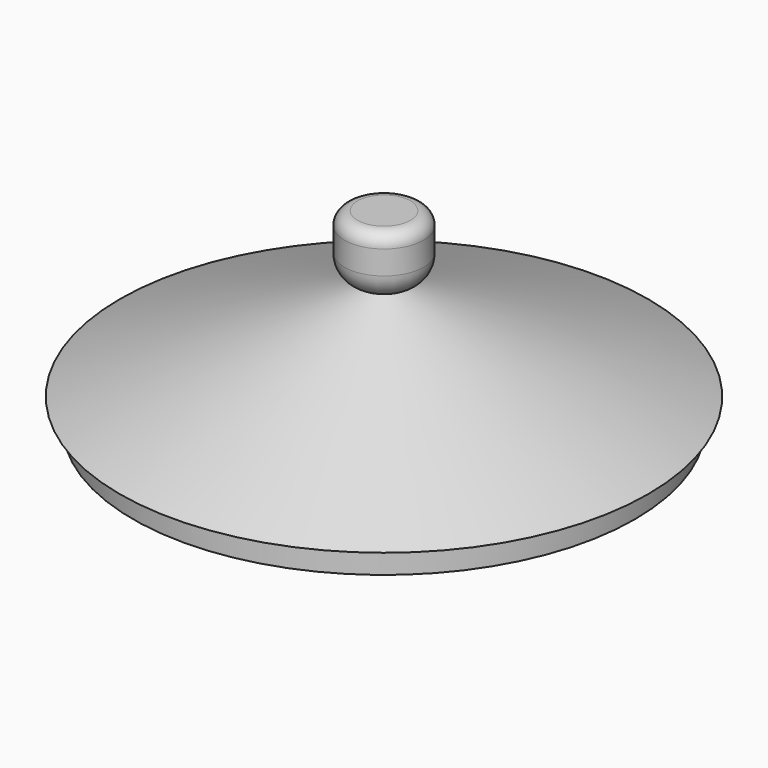
from build123d import *

# Parameters (mm, degrees)
F2_R      = 2.5
F0_R      = 50
F5_R      = 7.5
F6_DEPTH  = 12
F7_R      = 2.5
F8_R      = 4.99999
F9_R      = 47.5
F10_DEPTH = 5


# Not quite as in the source:
# - a fillet or chamfer is up to 0.001 mm smaller than in the source, because OpenCascade refuses the exact size


with BuildPart() as f3:
    # F2 (on offset) → F3 section 0
    with BuildSketch(Plane.XY.offset(19)):
        Circle(F2_R)
    # F0 (on Top) → F3 section 1
    with BuildSketch(Plane.XY):
        Circle(F0_R)
    loft()

    # F5 (on offset) → F6 (join)
    with BuildSketch(Plane.XY.offset(19)):
        Circle(F5_R)
    extrude(amount=F6_DEPTH)

    # F7
    f7_edges = [f3.edges().sort_by_distance(p)[0] for p in [
        (-7.5, 0, 31),
    ]]
    fillet(f7_edges, radius=F7_R)

    # F8 (radius 5 in the source; OpenCascade refuses exactly that, so slightly less here)
    f8_edges = [f3.edges().sort_by_distance(p)[0] for p in [
        (-7.5, 0, 19),
    ]]
    fillet(f8_edges, radius=F8_R)

    # F9 (on Top) → F10 (join)
    with BuildSketch(Plane.XY):
        Circle(F9_R)
    extrude(amount=-F10_DEPTH)


with BuildPart() as f4:
    # F2 (on offset) → F4 section 0
    with BuildSketch(Plane.XY.offset(19)):
        Circle(F2_R)
    # F0 (on Top) → F4 section 1
    with BuildSketch(Plane.XY):
        Circle(F0_R)
    loft()


solid = Compound([f3.part, f4.part])
